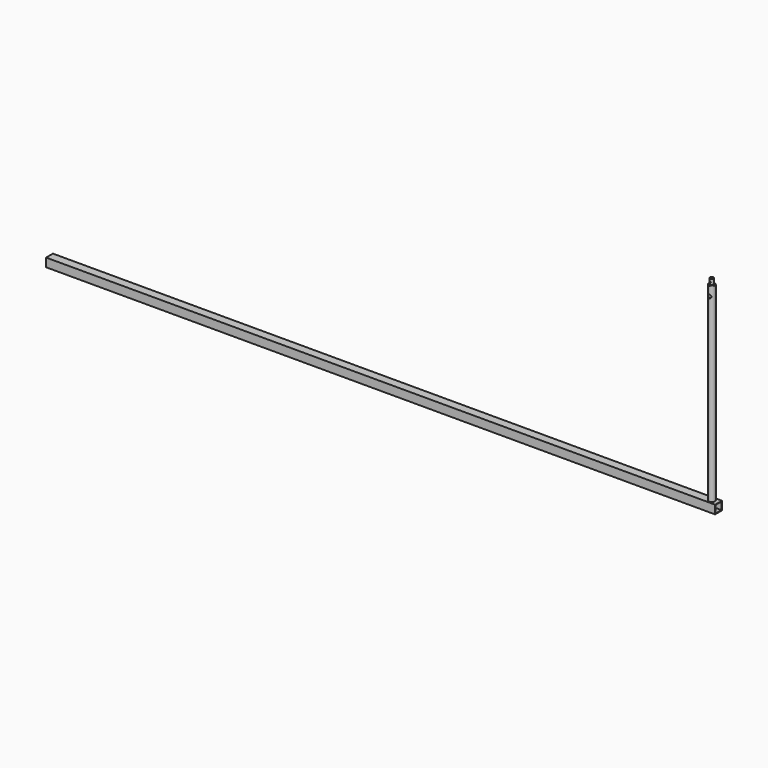
from build123d import *

# Parameters (mm, degrees)
F0_W      = 32
F0_H      = 32
F0_W_2    = 28
F0_H_2    = 28
F1_DEPTH  = 25
F2_DEPTH  = 2475
F3_R      = 11.55
F3_R_2    = 9.55
F4_DEPTH  = 710
F5_R      = 9.55
F6_DEPTH  = 25
F7_R      = 6.35
F8_DEPTH  = 21.5
F9_R      = 1.5
F10_DEPTH = 6.5
F11_R     = 9.55
F11_R_2   = 6.35
F12_DEPTH = 2
F13_R     = 6.35
F14_DEPTH = 25


with BuildPart() as f1:
    # F0 (on Right) → F1 (new body)
    with BuildSketch(Plane.YZ):
        Rectangle(F0_W, F0_H)
        Rectangle(F0_W_2, F0_H_2, mode=Mode.SUBTRACT)
    extrude(amount=F1_DEPTH)

    # F0 (on Right) → F2 (join)
    with BuildSketch(Plane.YZ):
        Rectangle(F0_W, F0_H)
        Rectangle(F0_W_2, F0_H_2, mode=Mode.SUBTRACT)
    extrude(amount=-F2_DEPTH)

    # F3 (on face) → F4 (join)
    with BuildSketch(Plane.XY.offset(16)):
        Circle(F3_R)
        Circle(F3_R_2, mode=Mode.SUBTRACT)
    extrude(amount=F4_DEPTH)

    # F13 (on Front) → F14 (cut)
    with BuildSketch(Plane.XZ):
        with Locations((0, 691)):
            Circle(F13_R)
    extrude(amount=F14_DEPTH, mode=Mode.SUBTRACT)


with BuildPart() as f6:
    # F5 (on face) → F6 (new body)
    with BuildSketch(Plane.XY.offset(726)):
        Circle(F5_R)
    extrude(amount=-F6_DEPTH)

    # F7 (on face) → F8 (join)
    with BuildSketch(Plane.XY.offset(726)):
        Circle(F7_R)
    extrude(amount=F8_DEPTH)

    # F9 (on Front) → F10 (cut, symmetric)
    with BuildSketch(Plane.XZ):
        with Locations((0, 735.5)):
            Circle(F9_R)
    extrude(amount=F10_DEPTH, both=True, mode=Mode.SUBTRACT)

    # F11 (on face) → F12 (join)
    with BuildSketch(Plane.XY.offset(726)):
        Circle(F11_R)
        Circle(F11_R_2, mode=Mode.SUBTRACT)
    extrude(amount=F12_DEPTH)


solid = Compound([f1.part, f6.part])
